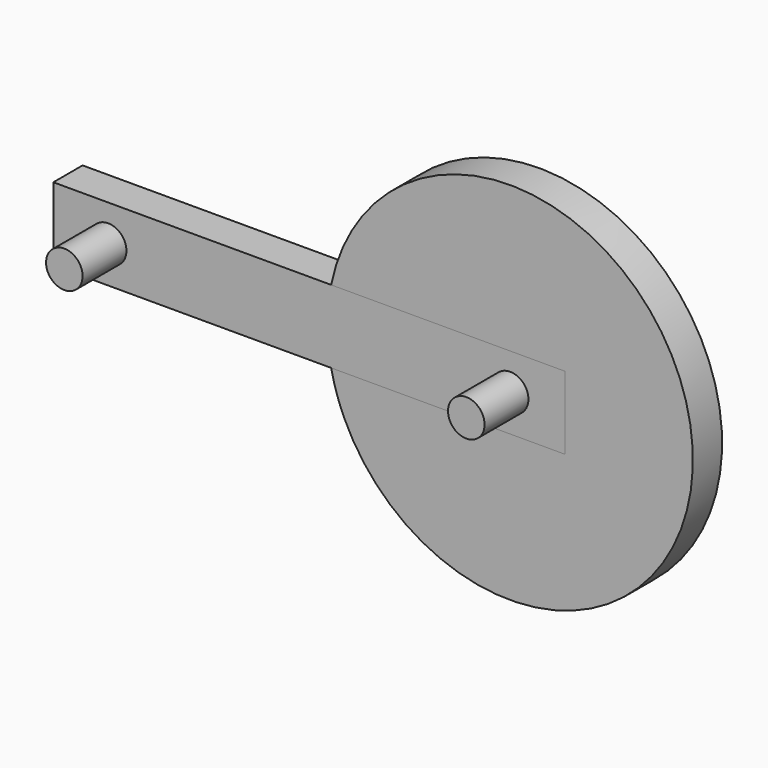
from build123d import *

# Parameters (mm, degrees)
F0_R     = 5
F1_DEPTH = 10
F2_DEPTH = 10
F3_DEPTH = 25


with BuildPart() as f1:
    # F0 (on Front) → F1 (new body)
    with BuildSketch(Plane.XZ):
        with BuildLine():
            ThreePointArc((-48.9897948557, -10), (-47.5316208531, -15.5159601403), (-45.4545454545, -20.8298895225))
            ThreePointArc((-45.4545454545, -20.8298895225), (10.6600358178, -48.8504210459), (50, 0))
            ThreePointArc((50, 0), (5.0254481003, 49.7468076503), (-48.9897948557, 10))
            Line((-48.9897948557, 10), (15, 10))
            Line((15, 10), (15, -10))
            Line((15, -10), (-48.9897948557, -10))
        make_face()
        with BuildLine():
            ThreePointArc((-49.9733265685, 1.6329824498), (-49.8222482499, -4.2123128242), (-48.9897948557, -10))
            Line((-48.9897948557, -10), (15, -10))
            Line((15, -10), (15, 10))
            Line((15, 10), (-48.9897948557, 10))
            ThreePointArc((-48.9897948557, 10), (-49.658096985, 5.8372428275), (-49.9733265685, 1.6329824498))
        make_face()
        Circle(F0_R, mode=Mode.SUBTRACT)
        with BuildLine():
            Line((-54.2726393539, -10), (-48.9897948557, -10))
            ThreePointArc((-48.9897948557, -10), (-49.8222482499, -4.2123128242), (-49.9733265685, 1.6329824498))
            ThreePointArc((-49.9733265685, 1.6329824498), (-52.5339055309, 0.9619130855), (-55, 0))
            ThreePointArc((-55, 0), (-57.5581280265, -1.3747285383), (-59.9218172427, -3.0619958092))
            Line((-59.9218172427, -3.0619958092), (-54.2726393539, -10))
        make_face()
    extrude(amount=F1_DEPTH)


with BuildPart() as f2:
    # F0 (on Front) → F2 (new body)
    with BuildSketch(Plane.XZ):
        with BuildLine():
            Line((-125, -10), (-54.2726393539, -10))
            Line((-54.2726393539, -10), (-59.9218172427, -3.0619958092))
            ThreePointArc((-59.9218172427, -3.0619958092), (-57.5581280265, -1.3747285383), (-55, 0))
            ThreePointArc((-55, 0), (-52.5339055309, 0.9619130855), (-49.9733265685, 1.6329824498))
            ThreePointArc((-49.9733265685, 1.6329824498), (-49.658096985, 5.8372428275), (-48.9897948557, 10))
            Line((-48.9897948557, 10), (-125, 10))
            Line((-125, 10), (-125, -10))
        make_face()
        with Locations((-110, 0)):
            Circle(F0_R, mode=Mode.SUBTRACT)
        with BuildLine():
            ThreePointArc((-49.9733265685, 1.6329824498), (-49.8222482499, -4.2123128242), (-48.9897948557, -10))
            Line((-48.9897948557, -10), (15, -10))
            Line((15, -10), (15, 10))
            Line((15, 10), (-48.9897948557, 10))
            ThreePointArc((-48.9897948557, 10), (-49.658096985, 5.8372428275), (-49.9733265685, 1.6329824498))
        make_face()
        Circle(F0_R, mode=Mode.SUBTRACT)
        with BuildLine():
            Line((-54.2726393539, -10), (-48.9897948557, -10))
            ThreePointArc((-48.9897948557, -10), (-49.8222482499, -4.2123128242), (-49.9733265685, 1.6329824498))
            ThreePointArc((-49.9733265685, 1.6329824498), (-52.5339055309, 0.9619130855), (-55, 0))
            ThreePointArc((-55, 0), (-57.5581280265, -1.3747285383), (-59.9218172427, -3.0619958092))
            Line((-59.9218172427, -3.0619958092), (-54.2726393539, -10))
        make_face()
        with Locations((-110, 0)):
            Circle(F0_R)
        Circle(F0_R)
    extrude(amount=F2_DEPTH)

    # F0 (on Front) → F3 (join)
    with BuildSketch(Plane.XZ):
        with Locations((-110, 0)):
            Circle(F0_R)
        Circle(F0_R)
    extrude(amount=F3_DEPTH)


solid = Compound([f1.part, f2.part])
